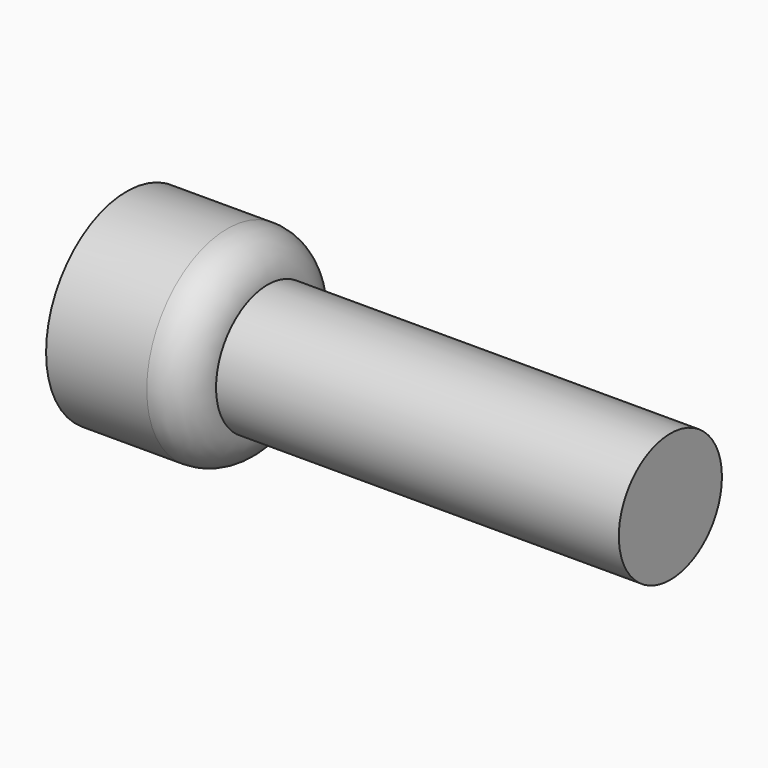
from build123d import *

# Parameters (mm, degrees)
F0_R      = 16
F1_DEPTH  = 100
F2_R      = 25
F3_DEPTH  = 35
F4_R      = 23
F5_DEPTH  = 10
F6_R      = 21
F7_DEPTH  = 2
F8_R      = 19
F9_DEPTH  = 2
F10_R     = 10
F12_DEPTH = 5


# Not quite as in the source:
# - a feature names something its author has since deleted; it is built from what else it names


with BuildPart() as f1:
    # F0 (on Right) → F1 (new body)
    with BuildSketch(Plane.YZ):
        Circle(F0_R)
    extrude(amount=F1_DEPTH)

    # F11 (on Top) → F12 (join)
    with BuildSketch(Plane.XY):
        with BuildLine():
            ThreePointArc((59.4952985912, 21.8782344051), (42.8892672062, 18.4997083247), (26.2832358212, 21.8782344051))
            Line((26.2832358212, 21.8782344051), (22.8892672062, 15.9997083247))
            Line((22.8892672062, 15.9997083247), (62.8892672062, 15.9997083247))
            Line((62.8892672062, 15.9997083247), (59.4952985912, 21.8782344051))
        make_face()
    extrude(amount=-F12_DEPTH)


with BuildPart() as f3:
    # F2 (on face) → F3 (new body)
    with BuildSketch(Plane(origin=(0, 0, 0), x_dir=(0, -1, 0), z_dir=(-1, 0, 0))):
        Circle(F2_R)
    extrude(amount=F3_DEPTH)

    # F4 (on face) → F5 (cut)
    with BuildSketch(Plane(origin=(-35, 0, 0), x_dir=(0, -1, 0), z_dir=(-1, 0, 0))):
        Circle(F4_R)
    extrude(amount=-F5_DEPTH, mode=Mode.SUBTRACT)

    # F6 (on face) → F7 (cut)
    with BuildSketch(Plane(origin=(-25, 0, 0), x_dir=(0, -1, 0), z_dir=(-1, 0, 0))):
        Circle(F6_R)
    extrude(amount=-F7_DEPTH, mode=Mode.SUBTRACT)

    # F8 (on face) → F9 (cut)
    with BuildSketch(Plane(origin=(-23, 0, 0), x_dir=(0, -1, 0), z_dir=(-1, 0, 0))):
        Circle(F8_R)
    extrude(amount=-F9_DEPTH, mode=Mode.SUBTRACT)

    # F10
    f10_edges = [f3.edges().sort_by_distance(p)[0] for p in [
        (0, 25, 0),
    ]]
    fillet(f10_edges, radius=F10_R)


solid = Compound([f1.part, f3.part])
